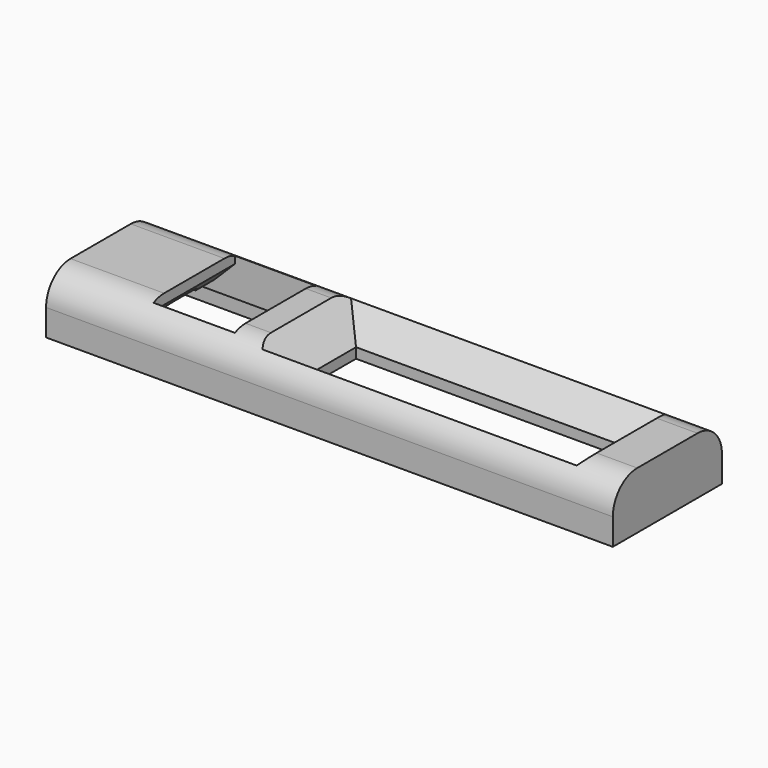
from build123d import *

# Parameters (mm, degrees)
F0_W          = 55.7
F0_H          = 13.4
F1_DEPTH      = 1.6
F2_W          = 55.7
F2_H          = 13.4
F2_W_2        = 26
F2_H_2        = 6
F3_DEPTH      = 4
F4_W          = 8
F4_H          = 10
F5_DEPTH      = 3
F6_T1_DEPTH   = 70.7
F7_W          = 6
F7_H          = 3.5
F8_DEPTH      = 10
F9_R          = 2
F10_T4_DEPTH  = 21.4300979278
F10_T10_DEPTH = 41.4300979278
F10_T16_DEPTH = 41.4300979278
F10_T22_DEPTH = 21.4300979278
F11_C1_SIZE   = 2
F11_C2_SIZE   = 2


# Not quite as in the source:
# - a fillet or chamfer that OpenCascade refuses, or shapes differently, is made with other operations: its cross-section is extruded or revolved along the edge and cut away or added


with BuildPart() as f1:
    # F0 (on Top) → F1 (new body)
    with BuildSketch(Plane.XY):
        with Locations((-20.85, 5.5)):
            Rectangle(F0_W, F0_H)
        Polygon((1, 0), (0, 0), (-47.5, 0), (-47.5, 11), (0, 11), (1, 11), align=None, mode=Mode.SUBTRACT)
    extrude(amount=F1_DEPTH)

    # F2 (on face) → F3 (join)
    with BuildSketch(Plane.XY.offset(1.6)):
        with Locations((-20.85, 5.5)):
            Rectangle(F2_W, F2_H)
        Polygon((-47.5, 0.5), (-47.5, 10.5), (-47.5, 11), (1, 11), (1, 0), (-47.5, 0), align=None, mode=Mode.SUBTRACT)
        Polygon((-47.5, 11), (-47.5, 10.5), (-31.5, 10.5), (-31.5, 0.5), (-47.5, 0.5), (-47.5, 0), (1, 0), (1, 11), align=None)
        with Locations((-13, 5.5)):
            Rectangle(F2_W_2, F2_H_2, mode=Mode.SUBTRACT)
    extrude(amount=F3_DEPTH)

    # F4 (on face) → F5 (join)
    with BuildSketch(Plane.XY.offset(5.6)):
        Polygon((-39.5, 12.2), (-48.7, 12.2), (-48.7, -1.2), (-39.5, -1.2), (-39.5, 0.5), (-47.5, 0.5), (-47.5, 10.5), (-39.5, 10.5), align=None)
        with Locations((-43.5, 5.5)):
            Rectangle(F4_W, F4_H)
    extrude(amount=-F5_DEPTH)

    # F6: fillet of radius 3 on 2 edges, made by hand

    # F6_s2 → F6_t1 (cut)
    with BuildSketch(Plane.YZ.offset(-56.2)):
        with BuildLine():
            ThreePointArc((12.2, 2.6), (11.3213203436, 4.7213203436), (9.2, 5.6))
            Line((9.2, 5.6), (12.2, 5.6))
            Line((12.2, 5.6), (12.2, 2.6))
        make_face()
        with BuildLine():
            ThreePointArc((1.8, 5.6), (-0.3213203436, 4.7213203436), (-1.2, 2.6))
            Line((-1.2, 2.6), (-1.2, 5.6))
            Line((-1.2, 5.6), (1.8, 5.6))
        make_face()
    extrude(amount=F6_T1_DEPTH, mode=Mode.SUBTRACT)

    # F7 (on face) → F8 (cut)
    with BuildSketch(Plane(origin=(-48.7, 0, 0), x_dir=(0, -1, 0), z_dir=(-1, 0, 0))):
        with Locations((-5.5, 1.75)):
            Rectangle(F7_W, F7_H)
    extrude(amount=-F8_DEPTH, mode=Mode.SUBTRACT)

    # F9
    f9_edges = [f1.edges().sort_by_distance(p)[0] for p in [
        (-44.1, 8.5, 3.5),
        (-44.1, 2.5, 3.5),
    ]]
    fillet(f9_edges, radius=F9_R)

    # F10: chamfer of 3 on 4 edges, made by hand


with BuildPart() as f10_tool2:
    # F10_s3 → F10_t4 (new body)
    with BuildSketch(Plane.XZ.offset(5.2150489639)):
        Polygon((-29, 5.6), (-26, 2.6), (-26, 5.6), align=None)
    extrude(amount=-F10_T4_DEPTH)

    split(bisect_by=Plane(origin=(0, 2.55, 2.55), x_dir=(1, 0, 0), z_dir=(0, 0.7071067812, 0.7071067812)), keep=Keep.TOP)

    split(bisect_by=Plane(origin=(0, 2.95, -2.95), x_dir=(1, 0, 0), z_dir=(0, -0.7071067812, 0.7071067812)), keep=Keep.TOP)


with BuildPart() as f1_1:
    add(f1.part)

    # F10_t1: cut F10_tool2
    add(f10_tool2.part, mode=Mode.SUBTRACT)


with BuildPart() as f10_tool8:
    # F10_s9 → F10_t10 (new body)
    with BuildSketch(Plane.YZ.offset(-33.7150489639)):
        Polygon((11.5, 5.6), (8.5, 2.6), (8.5, 5.6), align=None)
    extrude(amount=F10_T10_DEPTH)

    split(bisect_by=Plane(origin=(-11.7, 0, -11.7), x_dir=(0, 1, 0), z_dir=(0.7071067812, 0, 0.7071067812)), keep=Keep.TOP)

    split(bisect_by=Plane(origin=(-1.3, 0, 1.3), x_dir=(0, 1, 0), z_dir=(-0.7071067812, 0, 0.7071067812)), keep=Keep.TOP)


with BuildPart() as f1_2:
    add(f1_1.part)

    # F10_t7: cut F10_tool8
    add(f10_tool8.part, mode=Mode.SUBTRACT)


with BuildPart() as f10_tool14:
    # F10_s15 → F10_t16 (new body)
    with BuildSketch(Plane.YZ.offset(7.7150489639)):
        Polygon((-0.5, 5.6), (2.5, 2.6), (2.5, 5.6), align=None)
    extrude(amount=-F10_T16_DEPTH)

    split(bisect_by=Plane(origin=(-11.7, 0, -11.7), x_dir=(0, 1, 0), z_dir=(0.7071067812, 0, 0.7071067812)), keep=Keep.TOP)

    split(bisect_by=Plane(origin=(-1.3, 0, 1.3), x_dir=(0, 1, 0), z_dir=(-0.7071067812, 0, 0.7071067812)), keep=Keep.TOP)


with BuildPart() as f1_3:
    add(f1_2.part)

    # F10_t13: cut F10_tool14
    add(f10_tool14.part, mode=Mode.SUBTRACT)


with BuildPart() as f10_tool20:
    # F10_s21 → F10_t22 (new body)
    with BuildSketch(Plane.XZ.offset(-16.2150489639)):
        Polygon((3, 5.6), (0, 2.6), (0, 5.6), align=None)
    extrude(amount=F10_T22_DEPTH)

    split(bisect_by=Plane(origin=(0, 2.55, 2.55), x_dir=(1, 0, 0), z_dir=(0, 0.7071067812, 0.7071067812)), keep=Keep.TOP)

    split(bisect_by=Plane(origin=(0, 2.95, -2.95), x_dir=(1, 0, 0), z_dir=(0, -0.7071067812, 0.7071067812)), keep=Keep.TOP)


with BuildPart() as f1_4:
    add(f1_3.part)

    # F10_t19: cut F10_tool20
    add(f10_tool20.part, mode=Mode.SUBTRACT)

    # F11: chamfer of 2 on 3 edges, made by hand

    # F11_c1
    f11_c1_edges = [f1_4.edges().sort_by_distance(p)[0] for p in [
        (-31.5, 5.5, 1.6),
    ]]
    chamfer(f11_c1_edges, length=F11_C1_SIZE)

    # F11_c2
    f11_c2_edges = [f1_4.edges().sort_by_distance(p)[0] for p in [
        (-39.5, 9.3351646544, 2.6),
    ]]
    chamfer(f11_c2_edges, length=F11_C2_SIZE)


solid = f1_4.part
